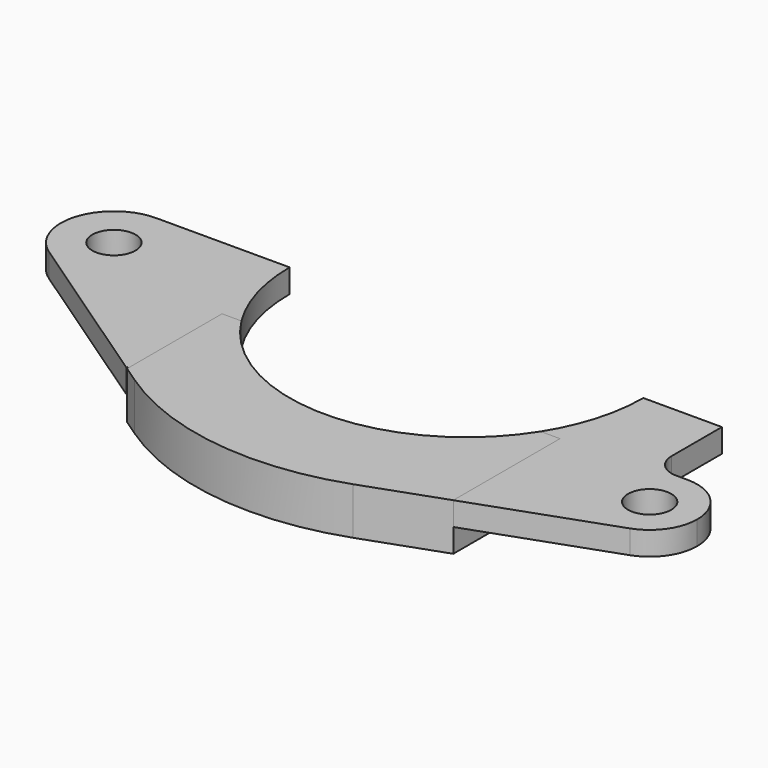
from build123d import *

# Parameters (mm, degrees)
F0_R     = 2.75
F1_DEPTH = 3
F2_DEPTH = 6


# Not quite as in the source:
# - a feature names something its author has since deleted; it is built from what else it names


with BuildPart() as f1:
    # F0 (on Top) → F1 (new body)
    with BuildSketch(Plane.XY):
        with BuildLine():
            ThreePointArc((-33.2160406839, -9.3244110423), (-34.0059545463, -5.8176503326), (-34.4267003209, -2.2477333057))
            ThreePointArc((-34.4267003209, -2.2477333057), (-36.7015374081, -0.5875004995), (-39.4558249578, 0))
            ThreePointArc((-39.4558249578, 0), (-45.9077806089, -4.7663749659), (-43.2479022167, -12.334142733))
            ThreePointArc((-43.2479022167, -12.334142733), (-37.5161243055, -13.215296697), (-33.2160406839, -9.3244110423))
        make_face()
        with Locations((-39.4558249578, -6.75)):
            Circle(F0_R, mode=Mode.SUBTRACT)
        with BuildLine():
            ThreePointArc((-21.6952147359, -26.8247582946), (-28.8162633149, -18.9703180935), (-33.2160406839, -9.3244110423))
            ThreePointArc((-33.2160406839, -9.3244110423), (-37.5161243055, -13.215296697), (-43.2479022167, -12.334142733))
            Line((-43.2479022167, -12.334142733), (-21.6914522522, -26.9726875554))
            Line((-21.6914522522, -26.9726875554), (-21.6952147359, -26.8247582946))
        make_face()
        with BuildLine():
            ThreePointArc((-32.7058249578, -6.75), (-33.1507043682, -4.3400302179), (-34.4267003209, -2.2477333057))
            ThreePointArc((-34.4267003209, -2.2477333057), (-34.0059545463, -5.8176503326), (-33.2160406839, -9.3244110423))
            ThreePointArc((-33.2160406839, -9.3244110423), (-32.8346074018, -8.0622416224), (-32.7058249578, -6.75))
        make_face()
        with BuildLine():
            ThreePointArc((-34.4267003209, -2.2477333057), (-34.4816702109, -1.1244640786), (-34.5, 0))
            Line((-34.5, 0), (-39.4558249578, 0))
            ThreePointArc((-39.4558249578, 0), (-36.7015374081, -0.5875004995), (-34.4267003209, -2.2477333057))
        make_face()
        with BuildLine():
            ThreePointArc((-19.0328663107, -12), (-21.6158447902, -6.2454186413), (-22.5, 0))
            Line((-22.5, 0), (-34.5, 0))
            ThreePointArc((-34.5, 0), (-34.4816702109, -1.1244640786), (-34.4267003209, -2.2477333057))
            ThreePointArc((-34.4267003209, -2.2477333057), (-33.1507043682, -4.3400302179), (-32.7058249578, -6.75))
            ThreePointArc((-32.7058249578, -6.75), (-32.8346074018, -8.0622416224), (-33.2160406839, -9.3244110423))
            ThreePointArc((-33.2160406839, -9.3244110423), (-28.8162633149, -18.9703180935), (-21.6952147359, -26.8247582946))
            ThreePointArc((-21.6952147359, -26.8247582946), (-21.5977495138, -26.9032937749), (-21.5, -26.9814751265))
            Line((-21.5, -26.9814751265), (-21.5, -12))
            Line((-21.5, -12), (-19.0328663107, -12))
        make_face()
    extrude(amount=-F1_DEPTH)


with BuildPart() as f1b:
    # F0 (on Top) → F1, piece 2 (new body)
    with BuildSketch(Plane.XY):
        with BuildLine():
            ThreePointArc((22.5, 0), (22.2485954613, -3.3541019663), (21.5, -6.6332495807))
            Line((21.5, -6.6332495807), (21.5, -12))
            Line((21.5, -12), (21.5, -26.9814751265))
            Line((21.5, -26.9814751265), (21.5, -28.9688625831))
            Line((21.5, -28.9688625831), (38.9781076545, -22.749936784))
            ThreePointArc((38.9781076545, -22.749936784), (30.9881581058, -18.0790487007), (36.95, -11))
            Line((36.95, -11), (35.5, -11))
            ThreePointArc((35.5, -11), (33.3786796564, -10.1213203436), (32.5, -8))
            Line((32.5, -8), (32.5, 0))
            Line((32.5, 0), (22.5, 0))
        make_face()
        with BuildLine():
            ThreePointArc((36.95, -11), (30.9881581058, -18.0790487007), (38.9781076545, -22.749936784))
            ThreePointArc((38.9781076545, -22.749936784), (41.8933061462, -20.5380115174), (43, -17.05))
            ThreePointArc((43, -17.05), (41.2279960262, -12.7720039738), (36.95, -11))
        make_face()
        with Locations((36.95, -17.05)):
            Circle(F0_R, mode=Mode.SUBTRACT)
        with BuildLine():
            ThreePointArc((21.5, -6.6332495807), (20.4433073488, -9.3979351266), (19.0328663107, -12))
            Line((19.0328663107, -12), (21.5, -12))
            Line((21.5, -12), (21.5, -6.6332495807))
        make_face()
    extrude(amount=-F1_DEPTH)


with BuildPart() as f2:
    # F0 (on Top) → F2 (new body)
    with BuildSketch(Plane.XY):
        with BuildLine():
            ThreePointArc((19.0328663107, -12), (0, -22.5), (-19.0328663107, -12))
            Line((-19.0328663107, -12), (-21.5, -12))
            Line((-21.5, -12), (-21.5, -26.9814751265))
            ThreePointArc((-21.5, -26.9814751265), (-20.4557349054, -27.7815210073), (-19.3817282119, -28.5411739688))
            ThreePointArc((-19.3817282119, -28.5411739688), (-4.3817701298, -34.220609149), (11.5652419965, -32.5037717436))
            ThreePointArc((11.5652419965, -32.5037717436), (16.7616078302, -30.1545768159), (21.5, -26.9814751265))
            Line((21.5, -26.9814751265), (21.5, -12))
            Line((21.5, -12), (19.0328663107, -12))
        make_face()
        with BuildLine():
            ThreePointArc((-19.3817282119, -28.5411739688), (-20.4557349054, -27.7815210073), (-21.5, -26.9814751265))
            Line((-21.5, -26.9814751265), (-21.5, -27.102698869))
            Line((-21.5, -27.102698869), (-19.3817282119, -28.5411739688))
        make_face()
        with BuildLine():
            Line((21.5, -28.9688625831), (21.5, -26.9814751265))
            ThreePointArc((21.5, -26.9814751265), (16.7616078302, -30.1545768159), (11.5652419965, -32.5037717436))
            Line((11.5652419965, -32.5037717436), (21.5, -28.9688625831))
        make_face()
    extrude(amount=-F2_DEPTH)


solid = Compound([f1.part, f1b.part, f2.part])
